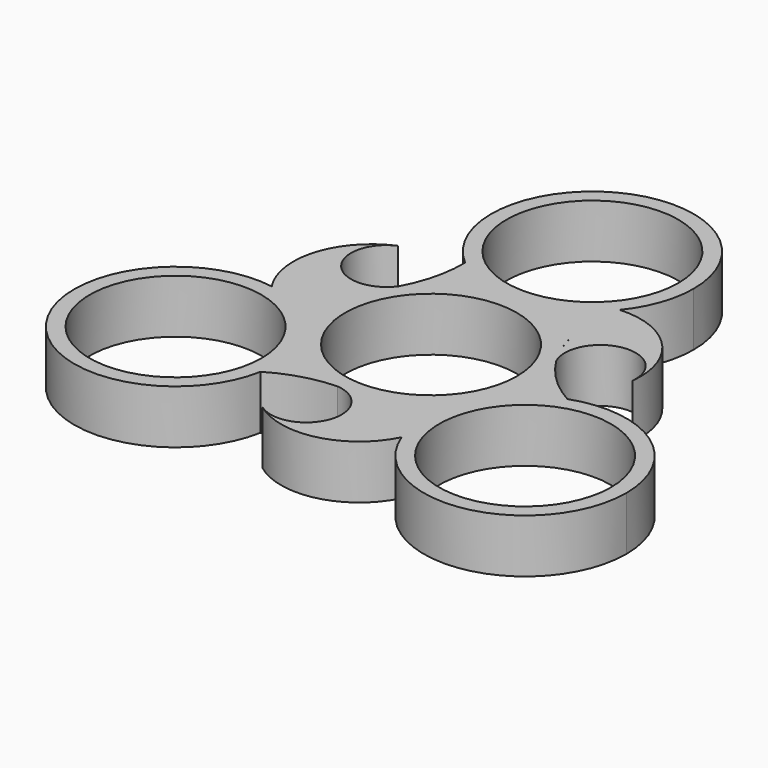
from build123d import *

# Parameters (mm, degrees)
F0_R     = 11.2
F1_DEPTH = 7
F3_DEPTH = 7


with BuildPart() as f1:
    # F0 (on Top) → F1 (new body)
    with BuildSketch(Plane.XY):
        with BuildLine():
            ThreePointArc((10.1597440205, 17.8761330961), (12.4166948314, 21.8239716806), (13.2, 26.3034459203))
            ThreePointArc((13.2, 26.3034459203), (-5.5373555744, 38.2858368855), (-8.5541959459, 16.2503005558))
            ThreePointArc((-8.5541959459, 16.2503005558), (-5.0829218379, 14.1213317529), (-1.12791098, 13.1517229602))
            ThreePointArc((-1.12791098, 13.1517229602), (0, 13.2), (1.12791098, 13.1517229602))
            ThreePointArc((1.12791098, 13.1517229602), (6.1182351733, 14.606984987), (10.1597440205, 17.8761330961))
        make_face()
        with Locations((0, 26.3034459203)):
            Circle(F0_R, mode=Mode.SUBTRACT)
        with BuildLine():
            ThreePointArc((-1.12791098, 13.1517229602), (-5.0829218379, 14.1213317529), (-8.5541959459, 16.2503005558))
            ThreePointArc((-8.5541959459, 16.2503005558), (-9.0756063849, 11.8077563343), (-10.7501080818, 7.6599723387))
            ThreePointArc((-10.7501080818, 7.6599723387), (-6.5430623893, 11.4642197541), (-1.12791098, 13.1517229602))
        make_face()
        with BuildLine():
            ThreePointArc((11.3058248826, 6.8130994213), (9.7913703879, 12.2470899677), (10.1597440205, 17.8761330961))
            ThreePointArc((10.1597440205, 17.8761330961), (6.1182351733, 14.606984987), (1.12791098, 13.1517229602))
            ThreePointArc((1.12791098, 13.1517229602), (6.9781074775, 11.204731859), (11.3058248826, 6.8130994213))
        make_face()
        with BuildLine():
            ThreePointArc((1.12791098, 13.1517229602), (0, 13.2), (-1.12791098, 13.1517229602))
            ThreePointArc((-1.12791098, 13.1517229602), (0, 13.1034459203), (1.12791098, 13.1517229602))
        make_face()
        with BuildLine():
            ThreePointArc((1.12791098, 13.1517229602), (0, 13.1034459203), (-1.12791098, 13.1517229602))
            ThreePointArc((-1.12791098, 13.1517229602), (-6.5430623893, 11.4642197541), (-10.7501080818, 7.6599723387))
            ThreePointArc((-10.7501080818, 7.6599723387), (-11.1373686058, 7.0132721384), (-11.5532296186, 6.3845818484))
            ThreePointArc((-11.5532296186, 6.3845818484), (-13.1926361713, 0.4408524163), (-11.9536816771, -5.5990619182))
            ThreePointArc((-11.9536816771, -5.5990619182), (-11.3479170441, -6.5517229602), (-10.825770697, -7.552661042))
            ThreePointArc((-10.825770697, -7.552661042), (-6.6567743469, -11.3985681247), (-1.2586765967, -13.1398528616))
            ThreePointArc((-1.2586765967, -13.1398528616), (-0.5049875326, -13.1518802131), (0.247404736, -13.1976812697))
            ThreePointArc((0.247404736, -13.1976812697), (6.2145286938, -11.6455842754), (10.825770697, -7.552661042))
            ThreePointArc((10.825770697, -7.552661042), (11.3479170441, -6.5517229602), (11.9536816771, -5.5990619182))
            ThreePointArc((11.9536816771, -5.5990619182), (12.8846536263, -2.8680482791), (13.2, 0))
            ThreePointArc((13.2, 0), (12.8987588115, 2.8039295858), (12.0087846785, 5.4798805229))
            ThreePointArc((12.0087846785, 5.4798805229), (11.6423561384, 6.1386080748), (11.3058248826, 6.8130994213))
            ThreePointArc((11.3058248826, 6.8130994213), (6.9781074775, 11.204731859), (1.12791098, 13.1517229602))
        make_face()
        Circle(F0_R, mode=Mode.SUBTRACT)
        with BuildLine():
            ThreePointArc((12.0087846785, 5.4798805229), (11.6763488687, 6.1565312552), (11.3058248826, 6.8130994213))
            ThreePointArc((11.3058248826, 6.8130994213), (11.6423561384, 6.1386080748), (12.0087846785, 5.4798805229))
        make_face()
        with BuildLine():
            ThreePointArc((-11.9536816771, -5.5990619182), (-13.1926361713, 0.4408524163), (-11.5532296186, 6.3845818484))
            ThreePointArc((-11.5532296186, 6.3845818484), (-15.5019762284, 2.35603051), (-20.5610573929, -0.1394701303))
            ThreePointArc((-20.5610573929, -0.1394701303), (-15.7091376581, -2.0049454071), (-11.9536816771, -5.5990619182))
        make_face()
        with BuildLine():
            ThreePointArc((18.3502710734, -0.7169992799), (14.7636201396, 1.955827517), (12.0087846785, 5.4798805229))
            ThreePointArc((12.0087846785, 5.4798805229), (12.8987588115, 2.8039295858), (13.2, 0))
            ThreePointArc((13.2, 0), (12.8846536263, -2.8680482791), (11.9536816771, -5.5990619182))
            ThreePointArc((11.9536816771, -5.5990619182), (14.7708929522, -2.6587264394), (18.3502710734, -0.7169992799))
        make_face()
        with BuildLine():
            ThreePointArc((-10.825770697, -7.552661042), (-11.3479170441, -6.5517229602), (-11.9536816771, -5.5990619182))
            ThreePointArc((-11.9536816771, -5.5990619182), (-11.43153533, -6.6), (-10.825770697, -7.552661042))
        make_face()
        with BuildLine():
            ThreePointArc((-10.825770697, -7.552661042), (-11.43153533, -6.6), (-11.9536816771, -5.5990619182))
            ThreePointArc((-11.9536816771, -5.5990619182), (-15.7091376581, -2.0049454071), (-20.5610573929, -0.1394701303))
            ThreePointArc((-20.5610573929, -0.1394701303), (-33.5968448072, -20.7163789966), (-9.7960751276, -15.533301276))
            ThreePointArc((-9.7960751276, -15.533301276), (-9.633719613, -14.3474278455), (-9.5794523741, -13.1517229602))
            ThreePointArc((-9.5794523741, -13.1517229602), (-9.8947987478, -10.283674681), (-10.825770697, -7.552661042))
        make_face()
        with Locations((-22.7794523741, -13.1517229602)):
            Circle(F0_R, mode=Mode.SUBTRACT)
        with BuildLine():
            ThreePointArc((35.9794523741, -13.1517229602), (30.3878295608, -2.3650368804), (18.3502710734, -0.7169992799))
            ThreePointArc((18.3502710734, -0.7169992799), (14.7708929522, -2.6587264394), (11.9536816771, -5.5990619182))
            ThreePointArc((11.9536816771, -5.5990619182), (11.43153533, -6.6), (10.825770697, -7.552661042))
            ThreePointArc((10.825770697, -7.552661042), (9.5909024848, -12.6020395799), (10.4013133724, -17.7366629658))
            ThreePointArc((10.4013133724, -17.7366629658), (25.1084613025, -26.1446332351), (35.9794523741, -13.1517229602))
        make_face()
        with Locations((22.7794523741, -13.1517229602)):
            Circle(F0_R, mode=Mode.SUBTRACT)
        with BuildLine():
            ThreePointArc((-1.2586765967, -13.1398528616), (-6.6567743469, -11.3985681247), (-10.825770697, -7.552661042))
            ThreePointArc((-10.825770697, -7.552661042), (-9.8947987478, -10.283674681), (-9.5794523741, -13.1517229602))
            ThreePointArc((-9.5794523741, -13.1517229602), (-9.633719613, -14.3474278455), (-9.7960751276, -15.533301276))
            ThreePointArc((-9.7960751276, -15.533301276), (-5.6880137547, -13.7635838512), (-1.2586765967, -13.1398528616))
        make_face()
        with BuildLine():
            ThreePointArc((10.825770697, -7.552661042), (11.43153533, -6.6), (11.9536816771, -5.5990619182))
            ThreePointArc((11.9536816771, -5.5990619182), (11.3479170441, -6.5517229602), (10.825770697, -7.552661042))
        make_face()
        with BuildLine():
            ThreePointArc((10.4013133724, -17.7366629658), (9.5909024848, -12.6020395799), (10.825770697, -7.552661042))
            ThreePointArc((10.825770697, -7.552661042), (6.2145286938, -11.6455842754), (0.247404736, -13.1976812697))
            ThreePointArc((0.247404736, -13.1976812697), (5.7106058405, -14.6031204777), (10.4013133724, -17.7366629658))
        make_face()
    extrude(amount=F1_DEPTH)

    # F2 (on Top) → F3 (join)
    with BuildSketch(Plane.XY):
        with BuildLine():
            ThreePointArc((12.2943036258, 4.9750674516), (15.5675466721, 11.6262977505), (20.9984593093, 6.580688525))
            ThreePointArc((20.9984593093, 6.580688525), (18.2353036168, 14.8413488661), (10.0971376523, 17.9467946291))
            ThreePointArc((10.0971376523, 17.9467946291), (9.9225536839, 11.2452805665), (12.2943036258, 4.9750674516))
        make_face()
        with BuildLine():
            ThreePointArc((-1.8386170143, -13.1347129876), (2.2848958678, -19.2950397679), (-4.8001862176, -21.4755434647))
            ThreePointArc((-4.8001862176, -21.4755434647), (3.735333336, -23.2129106109), (10.4938112391, -17.717775027))
            ThreePointArc((10.4938112391, -17.717775027), (4.7859075855, -14.1929896942), (-1.8386170143, -13.1347129876))
        make_face()
        with BuildLine():
            ThreePointArc((-10.4556866115, 8.159645536), (-17.85244254, 7.6687420174), (-16.1982730917, 14.8948549397))
            ThreePointArc((-16.1982730917, 14.8948549397), (-21.9706369528, 8.3715617448), (-20.5909488915, -0.2290196021))
            ThreePointArc((-20.5909488915, -0.2290196021), (-14.6756844073, 2.9411945739), (-10.4556866115, 8.159645536))
        make_face()
    extrude(amount=F3_DEPTH)


solid = f1.part
